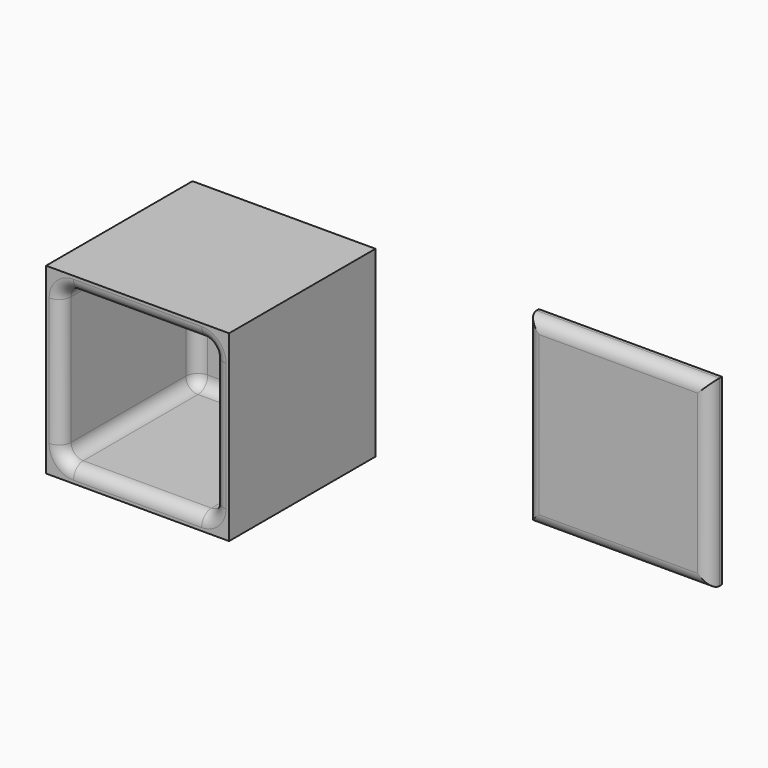
from build123d import *

# Parameters (mm, degrees)
F0_W         = 76.2
F0_H         = 76.2
F1_DEPTH     = 76.2
F2_W         = 63.5
F2_H         = 63.5
F3_DEPTH     = 69.85
F4_DEPTH     = 6.35
F5_R         = 5.08
F6_F1_R      = 5.08
F6_F2_R      = 5.08
F7_R         = 12.7
F8_DEPTH     = 5.08
F9_T1_DEPTH  = 53.34
F9_S5_W      = 5.08
F9_S5_H      = 5.08
F9_T6_DEPTH  = 5.08
F9_S11_W     = 5.08
F9_S11_H     = 5.08
F9_T12_DEPTH = 5.08
F9_S17_W     = 5.08
F9_S17_H     = 5.08
F9_T18_DEPTH = 5.08
F9_S23_W     = 5.08
F9_S23_H     = 5.08
F9_T24_DEPTH = 5.08


# Not quite as in the source:
# - a fillet or chamfer that OpenCascade refuses, or shapes differently, is made with other operations: its cross-section is extruded or revolved along the edge and cut away or added


with BuildPart() as f1:
    # F0 (on Front) → F1 (new body)
    with BuildSketch(Plane.XZ):
        Rectangle(F0_W, F0_H)
    extrude(amount=F1_DEPTH)

    # F2 (on face) → F3 (cut)
    with BuildSketch(Plane.XZ.offset(76.2)):
        Rectangle(F2_W, F2_H)
    extrude(amount=-F3_DEPTH, mode=Mode.SUBTRACT)

    # F6: fillet of radius 5.08 on 8 edges, made by hand

    # F6_f1
    f6_f1_edges = [f1.edges().sort_by_distance(p)[0] for p in [
        (31.75, -41.275, 31.75),
        (-31.75, -41.275, 31.75),
        (0, -6.35, 31.75),
        (-31.75, -41.275, -31.75),
        (31.75, -41.275, -31.75),
        (0, -6.35, -31.75),
    ]]
    fillet(f6_f1_edges, radius=F6_F1_R)

    # F6_f2
    f6_f2_edges = [f1.edges().sort_by_distance(p)[0] for p in [
        (0, -76.2, 31.75),
        (0, -76.2, -31.75),
        (-30.2621024484, -76.2, -30.2621024484),
        (30.2621024484, -76.2, -30.2621024484),
        (30.2621024484, -76.2, 30.2621024484),
        (-30.2621024484, -76.2, 30.2621024484),
    ]]
    fillet(f6_f2_edges, radius=F6_F2_R)

    # F9: fillet of radius 5.08 on 2 edges, made by hand

    # F9_s2 → F9_t1 (join)
    with BuildSketch(Plane.XY.offset(-26.67)):
        with BuildLine():
            ThreePointArc((-31.75, -11.43), (-30.2621024484, -7.8378975516), (-26.67, -6.35))
            Line((-26.67, -6.35), (-31.75, -6.35))
            Line((-31.75, -6.35), (-31.75, -11.43))
        make_face()
        with BuildLine():
            ThreePointArc((31.75, -11.43), (30.2621024484, -7.8378975516), (26.67, -6.35))
            Line((26.67, -6.35), (31.75, -6.35))
            Line((31.75, -6.35), (31.75, -11.43))
        make_face()
    extrude(amount=F9_T1_DEPTH)


with BuildPart() as f4:
    # F0 (on Front) → F4 (new body)
    with BuildSketch(Plane.XZ):
        with Locations((144.2514499441, 0)):
            Rectangle(F0_W, F0_H)
    extrude(amount=F4_DEPTH)

    # F5
    f5_edges = [f4.edges().sort_by_distance(p)[0] for p in [
        (144.25145, -6.35, -38.1),
        (182.35145, -6.35, 0),
        (144.25145, -6.35, 38.1),
        (106.15145, -6.35, 0),
    ]]
    fillet(f5_edges, radius=F5_R)


with BuildPart() as f8:
    # F7 (on Top) → F8 (new body)
    with BuildSketch(Plane.XY):
        with Locations((-62.8204271197, 35.6044583023)):
            Circle(F7_R)
    extrude(amount=F8_DEPTH)


with BuildPart() as f9_tool4:
    # F9_s5 → F9_t6 (new body)
    with BuildSketch(Plane.YZ.offset(26.67)):
        with Locations((-8.89, -29.21)):
            Rectangle(F9_S5_W, F9_S5_H)
    extrude(amount=F9_T6_DEPTH)

    # F9_s7 → F9_t8 (revolve, cut)
    with BuildSketch(Plane(origin=(26.67, -11.43, -26.67), x_dir=(0, -0.7071067812, 0.7071067812), z_dir=(0, 0.7071067812, 0.7071067812))):
        with BuildLine():
            ThreePointArc((0, -5.08), (5.08, 0), (0, 5.08))
            Line((0, 5.08), (0, -5.08))
        make_face()
    revolve(axis=Axis((26.67, -11.43, -26.67), (1, 0, 0)), mode=Mode.SUBTRACT)


with BuildPart() as f1_1:
    add(f1.part)

    # F9_t3: union F9_tool4
    add(f9_tool4.part)


with BuildPart() as f9_tool10:
    # F9_s11 → F9_t12 (new body)
    with BuildSketch(Plane.YZ.offset(26.67)):
        with Locations((-8.89, 29.21)):
            Rectangle(F9_S11_W, F9_S11_H)
    extrude(amount=F9_T12_DEPTH)

    # F9_s13 → F9_t14 (revolve, cut)
    with BuildSketch(Plane(origin=(26.67, -11.43, 26.67), x_dir=(0, -0.7071067812, -0.7071067812), z_dir=(0, -0.7071067812, 0.7071067812))):
        with BuildLine():
            ThreePointArc((0, -5.08), (5.08, 0), (0, 5.08))
            Line((0, 5.08), (0, -5.08))
        make_face()
    revolve(axis=Axis((26.67, -11.43, 26.67), (1, 0, 0)), mode=Mode.SUBTRACT)


with BuildPart() as f1_2:
    add(f1_1.part)

    # F9_t9: union F9_tool10
    add(f9_tool10.part)


with BuildPart() as f9_tool16:
    # F9_s17 → F9_t18 (new body)
    with BuildSketch(Plane.YZ.offset(-26.67)):
        with Locations((-8.89, 29.21)):
            Rectangle(F9_S17_W, F9_S17_H)
    extrude(amount=-F9_T18_DEPTH)

    # F9_s19 → F9_t20 (revolve, cut)
    with BuildSketch(Plane(origin=(-26.67, -11.43, 26.67), x_dir=(0, -0.7071067812, -0.7071067812), z_dir=(0, 0.7071067812, -0.7071067812))):
        with BuildLine():
            ThreePointArc((0, -5.08), (5.08, 0), (0, 5.08))
            Line((0, 5.08), (0, -5.08))
        make_face()
    revolve(axis=Axis((-26.67, -11.43, 26.67), (-1, 0, 0)), mode=Mode.SUBTRACT)


with BuildPart() as f1_3:
    add(f1_2.part)

    # F9_t15: union F9_tool16
    add(f9_tool16.part)


with BuildPart() as f9_tool22:
    # F9_s23 → F9_t24 (new body)
    with BuildSketch(Plane.YZ.offset(-26.67)):
        with Locations((-8.89, -29.21)):
            Rectangle(F9_S23_W, F9_S23_H)
    extrude(amount=-F9_T24_DEPTH)

    # F9_s25 → F9_t26 (revolve, cut)
    with BuildSketch(Plane(origin=(-26.67, -11.43, -26.67), x_dir=(0, -0.7071067812, 0.7071067812), z_dir=(0, -0.7071067812, -0.7071067812))):
        with BuildLine():
            ThreePointArc((0, -5.08), (5.08, 0), (0, 5.08))
            Line((0, 5.08), (0, -5.08))
        make_face()
    revolve(axis=Axis((-26.67, -11.43, -26.67), (-1, 0, 0)), mode=Mode.SUBTRACT)


with BuildPart() as f1_4:
    add(f1_3.part)

    # F9_t21: union F9_tool22
    add(f9_tool22.part)


solid = Compound([f4.part, f8.part, f1_4.part])
